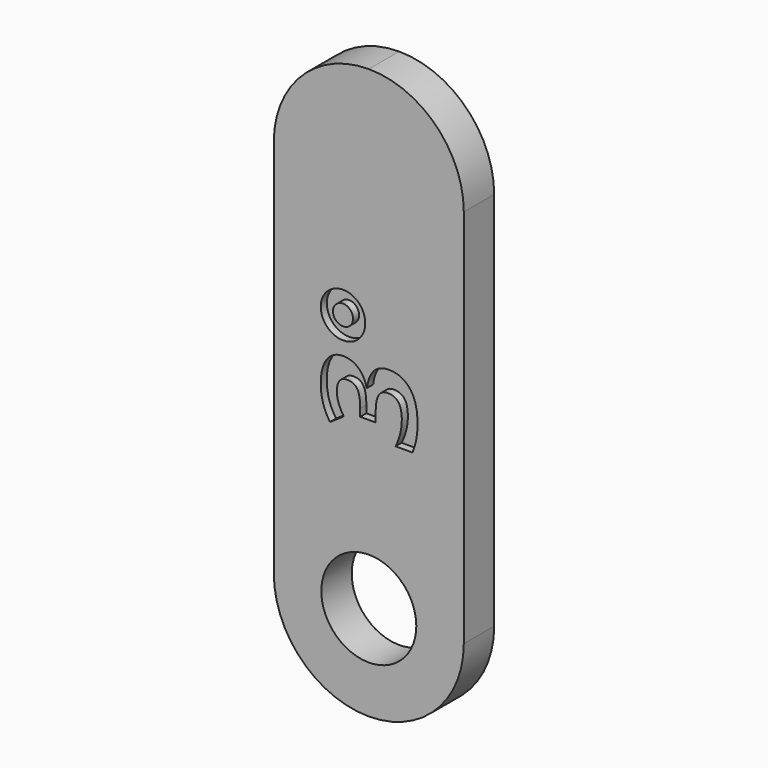
from build123d import *

# Parameters (mm, degrees)
F0_W         = 12.7
F0_H         = 38.1
F0_R         = 3.175
F1_DEPTH     = 2.54
F2_R         = 6.34999
F3_TEXT_SIZE = 8.8194444444
F4_DEPTH     = 0.508


# Not quite as in the source:
# - a fillet or chamfer is up to 0.001 mm smaller than in the source, because OpenCascade refuses the exact size
# - Text() gives the source's letters only with a copy of the font that has no kerning and outlines rounded to 1/6400 em; it was checked with that copy


with BuildPart() as f1:
    # F0 (on Front) → F1 (new body)
    with BuildSketch(Plane.XZ):
        with Locations((6.35, 19.05)):
            Rectangle(F0_W, F0_H)
        with Locations((6.35, 6.35)):
            Circle(F0_R, mode=Mode.SUBTRACT)
    extrude(amount=F1_DEPTH)

    # F2 (radius 6.35 in the source; OpenCascade refuses exactly that, so slightly less here)
    f2_edges = [f1.edges().sort_by_distance(p)[0] for p in [
        (12.7, -1.27, 0),
        (0, -1.27, 0),
        (12.7, -1.27, 38.1),
        (0, -1.27, 38.1),
    ]]
    fillet(f2_edges, radius=F2_R)

    # F3 (on face) → F4 (cut)
    with BuildSketch(Plane.XZ.offset(2.54)):
        with Locations(Location((9.525, 16.1464735243), (0, 0, 90))):
            Text('3°', F3_TEXT_SIZE, font='Open Sans', font_style=FontStyle.BOLD, text_align=(TextAlign.LEFT, TextAlign.BOTTOM))
    extrude(amount=-F4_DEPTH, mode=Mode.SUBTRACT)


solid = f1.part
